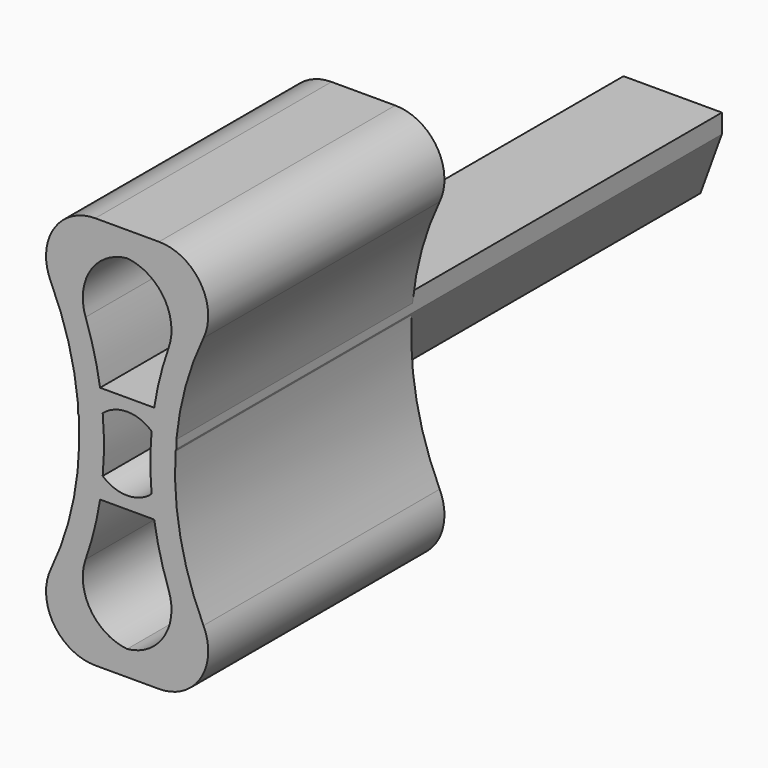
from build123d import *

# Parameters (mm, degrees)
F1_DEPTH      = 25.4
F1_DEPTH_BACK = 12.7
F2_T1_DEPTH   = 38.1
F2_T3_DEPTH   = 96.9143148495
F3_W          = 12.7
F3_H          = 12.7
F3_R          = 4.7625
F4_DEPTH      = 25.4
F5_W          = 12.7
F5_H          = 12.7
F6_DEPTH      = 12.7
F6_DEPTH_BACK = 12.7
F7_W          = 63.5
F7_H          = 10.0732017308
F8_DEPTH      = 6.35
F9_SIZE2      = 2.7734531851
F9_SIZE       = 7.62
F9_2_SIZE2    = 2.7734531851
F9_2_SIZE     = 7.62


# Not quite as in the source:
# - a fillet or chamfer that OpenCascade refuses, or shapes differently, is made with other operations: its cross-section is extruded or revolved along the edge and cut away or added


with BuildPart() as f1:
    # F0 (on Front) → F1 (new body, two sides)
    with BuildSketch(Plane.XZ) as f1_sk:
        with BuildLine():
            Line((15.875, 25.4), (-15.875, 25.4))
            ThreePointArc((-15.875, 25.4), (-6.1730633142, 0), (-15.875, -25.4))
            Line((-15.875, -25.4), (15.875, -25.4))
            ThreePointArc((15.875, -25.4), (6.1730633142, 0), (15.875, 25.4))
        make_face()
        with BuildLine():
            ThreePointArc((-9.4926809127, -22.225), (-2.9980633142, 0), (-9.4926809127, 22.225))
            Line((-9.4926809127, 22.225), (9.4926809127, 22.225))
            ThreePointArc((9.4926809127, 22.225), (2.9980633142, 0), (9.4926809127, -22.225))
            Line((9.4926809127, -22.225), (-9.4926809127, -22.225))
        make_face(mode=Mode.SUBTRACT)
    extrude(amount=F1_DEPTH)
    extrude(f1_sk.sketch, amount=-F1_DEPTH_BACK)

    # F2: fillet of radius 6.35 on 8 edges, made by hand

    # F2_s2 → F2_t1 (join)
    with BuildSketch(Plane.XZ.offset(-12.7)):
        with BuildLine():
            ThreePointArc((-0.6282172911, 22.225), (4.5565359978, 19.5411742094), (5.3586201229, 13.7583333333))
            ThreePointArc((5.3586201229, 13.7583333333), (7.1832676704, 18.1100161264), (9.4926809127, 22.225))
            Line((9.4926809127, 22.225), (-0.6282172911, 22.225))
        make_face()
        with BuildLine():
            ThreePointArc((-0.6282172911, -22.225), (4.5565359978, -19.5411742094), (5.3586201229, -13.7583333333))
            ThreePointArc((5.3586201229, -13.7583333333), (7.1832676704, -18.1100161264), (9.4926809127, -22.225))
            Line((9.4926809127, -22.225), (-0.6282172911, -22.225))
        make_face()
        with BuildLine():
            ThreePointArc((0.6282172911, 22.225), (-4.5565359978, 19.5411742094), (-5.3586201229, 13.7583333333))
            ThreePointArc((-5.3586201229, 13.7583333333), (-7.1832676704, 18.1100161264), (-9.4926809127, 22.225))
            Line((-9.4926809127, 22.225), (0.6282172911, 22.225))
        make_face()
        with BuildLine():
            ThreePointArc((-5.3586201229, -13.7583333333), (-4.5565359978, -19.5411742094), (0.6282172911, -22.225))
            Line((0.6282172911, -22.225), (-9.4926809127, -22.225))
            ThreePointArc((-9.4926809127, -22.225), (-7.1832676704, -18.1100161264), (-5.3586201229, -13.7583333333))
        make_face()
    extrude(amount=F2_T1_DEPTH)

    # F2_s4 → F2_t3 (cut)
    with BuildSketch(Plane.XZ.offset(-42.1071574247)):
        with BuildLine():
            ThreePointArc((-4.1121370301, 25.4), (-9.4788665476, 22.4442177723), (-9.8494122136, 16.3285714286))
            ThreePointArc((-9.8494122136, 16.3285714286), (-12.5364180191, 21.0806865498), (-15.875, 25.4))
            Line((-15.875, 25.4), (-4.1121370301, 25.4))
        make_face()
        with BuildLine():
            ThreePointArc((-9.8494122136, -16.3285714286), (-9.4788665476, -22.4442177723), (-4.1121370301, -25.4))
            Line((-4.1121370301, -25.4), (-15.875, -25.4))
            ThreePointArc((-15.875, -25.4), (-12.5364180191, -21.0806865498), (-9.8494122136, -16.3285714286))
        make_face()
        with BuildLine():
            ThreePointArc((4.1121370301, 25.4), (9.4788665476, 22.4442177723), (9.8494122136, 16.3285714286))
            ThreePointArc((9.8494122136, 16.3285714286), (12.5364180191, 21.0806865498), (15.875, 25.4))
            Line((15.875, 25.4), (4.1121370301, 25.4))
        make_face()
        with BuildLine():
            ThreePointArc((9.8494122136, -16.3285714286), (9.4788665476, -22.4442177723), (4.1121370301, -25.4))
            Line((4.1121370301, -25.4), (15.875, -25.4))
            ThreePointArc((15.875, -25.4), (12.5364180191, -21.0806865498), (9.8494122136, -16.3285714286))
        make_face()
    extrude(amount=F2_T3_DEPTH, mode=Mode.SUBTRACT)

    # F3 (on Front) → F4 (join)
    with BuildSketch(Plane.XZ):
        Rectangle(F3_W, F3_H)
        Circle(F3_R, mode=Mode.SUBTRACT)
    extrude(amount=F4_DEPTH)

    # F5 (on Front) → F6 (join, two sides)
    with BuildSketch(Plane.XZ) as f6_sk:
        Rectangle(F5_W, F5_H)
    extrude(amount=-F6_DEPTH)
    extrude(f6_sk.sketch, amount=F6_DEPTH_BACK)

    # F7 (on Right) → F8 (join, symmetric)
    with BuildSketch(Plane.YZ):
        with Locations((30.847759068, 0)):
            Rectangle(F7_W, F7_H)
    extrude(amount=F8_DEPTH, both=True)

    # F9
    f9_edges = [f1.edges().sort_by_distance(p)[0] for p in [
        (6.35, 37.64888, -5.036601),
    ]]
    f9_side = f1.faces().sort_by_distance((6.35, 21.926607, 0))[0]
    chamfer(f9_edges, length=F9_SIZE, length2=F9_SIZE2, reference=f9_side)

    # F9#2
    f9_2_edges = [f1.edges().sort_by_distance(p)[0] for p in [
        (-6.35, 37.64888, -5.036601),
    ]]
    f9_2_side = f1.faces().sort_by_distance((-6.35, 21.926607, 0))[0]
    chamfer(f9_2_edges, length=F9_2_SIZE, length2=F9_2_SIZE2, reference=f9_2_side)


solid = f1.part
